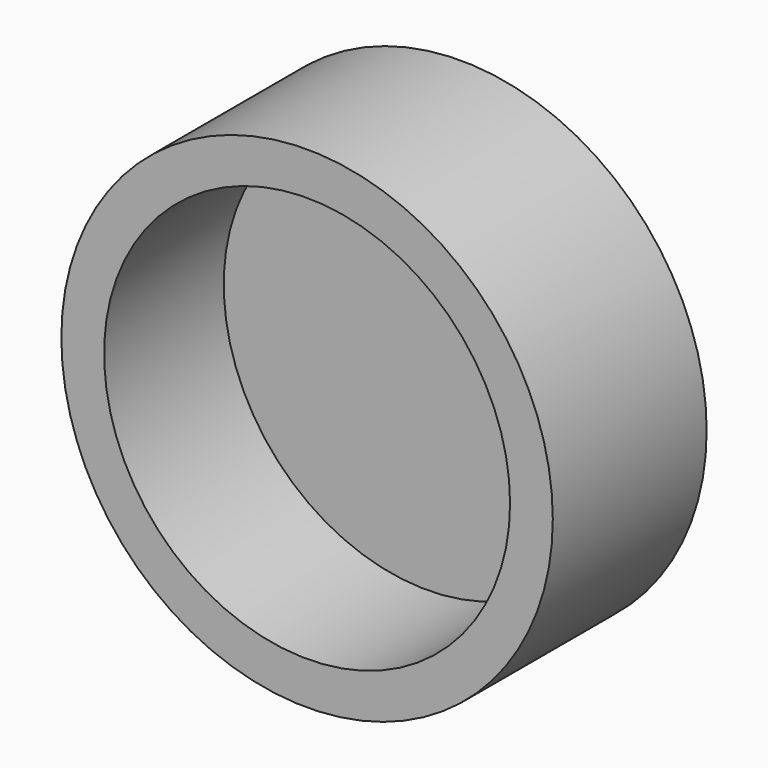
from build123d import *

# Parameters (mm, degrees)
F0_R     = 73.025
F1_DEPTH = 57.15
F2_DEPTH = 12.7


# Not quite as in the source:
# - ends of sketch curves that miss each other by under 0.0002 mm in the source are joined
# - the program builds the solid bodies; features that only make, move or delete a surface that nothing else refers to are left out


with BuildPart() as f1:
    # F0 (on Front) → F1 (new body)
    with BuildSketch(Plane.XZ):
        Circle(F0_R)
        with BuildLine():
            ThreePointArc((-60.325, 0), (0, 60.325), (60.325, 0))
            ThreePointArc((60.325, 0), (0, -60.325), (-60.325, 0))
        make_face(mode=Mode.SUBTRACT)
    extrude(amount=F1_DEPTH)

    # F0 (on Front) → F2 (join)
    with BuildSketch(Plane.XZ):
        with BuildLine():
            Line((-60.325, -1.5561e-06), (60.325, -1.5561e-06))
            ThreePointArc((60.325, -1.5561e-06), (0, 60.325), (-60.325, -1.5561e-06))
        make_face()
        with BuildLine():
            ThreePointArc((-60.325, 0), (0, -60.325), (60.325, 0))
            Line((60.325, 0), (-60.325, 0))
        make_face()
    extrude(amount=F2_DEPTH)


solid = f1.part
